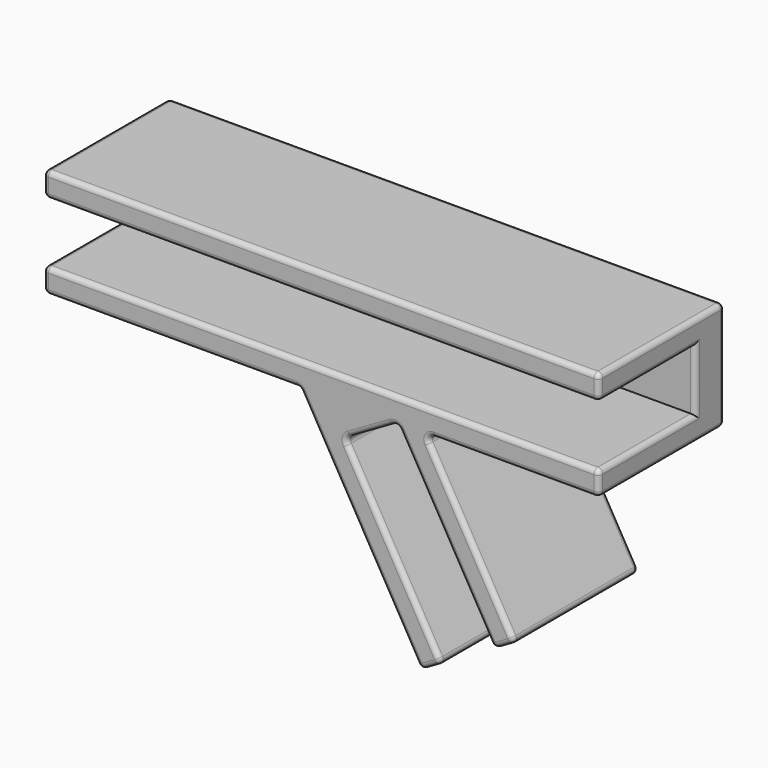
from build123d import *

# Parameters (mm, degrees)
F1_DEPTH      = 12.7
F0_W          = 58.42
F0_H          = 2.54
F0_H_2        = 6.35
F2_DEPTH      = 3.81
F4_T1_DEPTH   = 16.51
F4_T3_DEPTH   = 57.404
F4_T5_DEPTH   = 12.192
F4_T7_DEPTH   = 13.97
F4_T9_DEPTH   = 19.05
F4_T11_DEPTH  = 12.192
F4_T13_DEPTH  = 1.524
F4_T15_DEPTH  = 15.494
F4_T17_DEPTH  = 3.302
F4_T19_DEPTH  = 6.35
F4_T21_DEPTH  = 3.302
F4_T23_DEPTH  = 3.302
F4_T25_DEPTH  = 19.177
F4_T27_DEPTH  = 5.08
F4_T29_DEPTH  = 19.177
F4_T31_DEPTH  = 6.35
F4_S35_W      = 0.508
F4_S35_H      = 0.508
F4_T36_DEPTH  = 0.508
F4_S41_W      = 0.508
F4_S41_H      = 0.508
F4_T42_DEPTH  = 0.508
F4_S47_W      = 0.508
F4_S47_H      = 0.508
F4_T48_DEPTH  = 0.508
F4_S53_W      = 0.508
F4_S53_H      = 0.508
F4_T54_DEPTH  = 0.508
F4_S59_W      = 0.508
F4_S59_H      = 0.508
F4_T60_DEPTH  = 0.508
F4_S65_W      = 0.508
F4_S65_H      = 0.508
F4_T66_DEPTH  = 0.508
F4_S71_W      = 0.508
F4_S71_H      = 0.508
F4_T72_DEPTH  = 0.508
F4_S77_W      = 0.508
F4_S77_H      = 0.508
F4_T78_DEPTH  = 0.508
F4_S83_W      = 0.508
F4_S83_H      = 0.508
F4_T84_DEPTH  = 0.508
F4_S89_W      = 0.508
F4_S89_H      = 0.508
F4_T90_DEPTH  = 0.508
F4_T94_ANGLE  = 90
F4_T96_ANGLE  = 90
F4_T101_DEPTH = 13.462
F4_T105_DEPTH = 7.62
F4_T112_DEPTH = 13.462
F4_T116_DEPTH = 7.62
F4_T123_DEPTH = 13.462
F4_T127_DEPTH = 7.62
F4_T134_DEPTH = 7.62
F4_T138_DEPTH = 13.462
F4_T145_DEPTH = 13.462
F4_T149_DEPTH = 7.62
F4_T156_DEPTH = 13.462
F4_T160_DEPTH = 7.62
F4_T163_DEPTH = 26.130035698
F4_T165_DEPTH = 24.5987060633
F4_T167_DEPTH = 17.4130046129
F4_T169_DEPTH = 16.9025614013
F4_T174_DEPTH = 0.508
F4_S179_W     = 0.508
F4_S179_H     = 0.508
F4_T180_DEPTH = 0.508
F4_S185_W     = 0.508
F4_S185_H     = 0.508
F4_T186_DEPTH = 0.508
F4_T192_DEPTH = 0.508
F4_S197_W     = 0.508
F4_S197_H     = 0.508
F4_T198_DEPTH = 0.508
F4_T204_DEPTH = 0.508
F4_T210_DEPTH = 0.508
F4_S215_W     = 0.508
F4_S215_H     = 0.508
F4_T216_DEPTH = 0.508
F4_T220_ANGLE = 60
F4_T222_ANGLE = 120
F4_T224_ANGLE = 120
F4_T226_ANGLE = 60


# Not quite as in the source:
# - a fillet or chamfer that OpenCascade refuses, or shapes differently, is made with other operations: its cross-section is extruded or revolved along the edge and cut away or added


with BuildPart() as f1:
    # F0 (on Front) → F1 (new body)
    with BuildSketch(Plane.XZ):
        with BuildLine():
            Line((29.21, -5.715), (29.21, -3.175))
            Line((29.21, -3.175), (-29.21, -3.175))
            Line((-29.21, -3.175), (-29.21, -5.715))
            Line((-29.21, -5.715), (-2.2786703653, -5.715))
            Line((-2.2786703653, -5.715), (10.4213296347, -27.7120452561))
            Line((10.4213296347, -27.7120452561), (12.6210341604, -26.4420452561))
            Line((12.6210341604, -26.4420452561), (2.7785341604, -9.3943351826))
            ThreePointArc((2.7785341604, -9.3943351826), (2.7150973921, -8.912485089), (3.0109602918, -8.5269090512))
            Line((3.0109602918, -8.5269090512), (7.410369343, -5.9869090512))
            ThreePointArc((7.410369343, -5.9869090512), (7.8922194366, -5.9234722829), (8.2777954744, -6.2193351826))
            Line((8.2777954744, -6.2193351826), (18.1202954744, -23.2670452561))
            Line((18.1202954744, -23.2670452561), (20.32, -21.9970452561))
            Line((20.32, -21.9970452561), (10.9195567884, -5.715))
            Line((10.9195567884, -5.715), (29.21, -5.715))
        make_face()
    extrude(amount=F1_DEPTH)



with BuildPart() as f1b:
    # F0 (on Front) → F1, piece 2 (new body)
    with BuildSketch(Plane.XZ):
        with Locations((0, 4.445)):
            Rectangle(F0_W, F0_H)
    extrude(amount=F1_DEPTH)


with BuildPart() as f1_1:
    add(f1.part)

    add(f1b.part)  # F2 merges F1b
    # F0 (on Front) → F2 (join)
    with BuildSketch(Plane.XZ):
        with Locations((0, 4.445)):
            Rectangle(F0_W, F0_H)
        Rectangle(F0_W, F0_H_2)
        with BuildLine():
            Line((12.6210341604, -26.4420452561), (18.1202954744, -23.2670452561))
            Line((18.1202954744, -23.2670452561), (8.2777954744, -6.2193351826))
            ThreePointArc((8.2777954744, -6.2193351826), (7.8922194366, -5.9234722829), (7.410369343, -5.9869090512))
            Line((7.410369343, -5.9869090512), (3.0109602918, -8.5269090512))
            ThreePointArc((3.0109602918, -8.5269090512), (2.7150973921, -8.912485089), (2.7785341604, -9.3943351826))
            Line((2.7785341604, -9.3943351826), (12.6210341604, -26.4420452561))
        make_face()
        with BuildLine():
            Line((29.21, -5.715), (29.21, -3.175))
            Line((29.21, -3.175), (-29.21, -3.175))
            Line((-29.21, -3.175), (-29.21, -5.715))
            Line((-29.21, -5.715), (-2.2786703653, -5.715))
            Line((-2.2786703653, -5.715), (10.4213296347, -27.7120452561))
            Line((10.4213296347, -27.7120452561), (12.6210341604, -26.4420452561))
            Line((12.6210341604, -26.4420452561), (2.7785341604, -9.3943351826))
            ThreePointArc((2.7785341604, -9.3943351826), (2.7150973921, -8.912485089), (3.0109602918, -8.5269090512))
            Line((3.0109602918, -8.5269090512), (7.410369343, -5.9869090512))
            ThreePointArc((7.410369343, -5.9869090512), (7.8922194366, -5.9234722829), (8.2777954744, -6.2193351826))
            Line((8.2777954744, -6.2193351826), (18.1202954744, -23.2670452561))
            Line((18.1202954744, -23.2670452561), (20.32, -21.9970452561))
            Line((20.32, -21.9970452561), (10.9195567884, -5.715))
            Line((10.9195567884, -5.715), (29.21, -5.715))
        make_face()
    extrude(amount=-F2_DEPTH)

    # F3: union 

    # F4: fillet of radius 0.508 on 43 edges, made by hand

    # F4_s2 → F4_t1 (join)
    with BuildSketch(Plane.XZ.offset(-3.81)):
        with BuildLine():
            ThreePointArc((11.7994385987, -5.715), (11.3594976935, -5.969), (11.3594976935, -6.477))
            Line((11.3594976935, -6.477), (10.9195567884, -5.715))
            Line((10.9195567884, -5.715), (11.7994385987, -5.715))
        make_face()
        with BuildLine():
            ThreePointArc((-2.1320233969, -5.969), (-2.317964302, -5.7830590949), (-2.571964302, -5.715))
            Line((-2.571964302, -5.715), (-2.2786703653, -5.715))
            Line((-2.2786703653, -5.715), (-2.1320233969, -5.969))
        make_face()
    extrude(amount=F4_T1_DEPTH)

    # F4_s4 → F4_t3 (cut)
    with BuildSketch(Plane.YZ.offset(-28.702)):
        with BuildLine():
            ThreePointArc((3.302, 5.715), (3.6612102448, 5.5662102448), (3.81, 5.207))
            Line((3.81, 5.207), (3.81, 5.715))
            Line((3.81, 5.715), (3.302, 5.715))
        make_face()
        with BuildLine():
            ThreePointArc((-12.7, 5.207), (-12.5512102448, 5.5662102448), (-12.192, 5.715))
            Line((-12.192, 5.715), (-12.7, 5.715))
            Line((-12.7, 5.715), (-12.7, 5.207))
        make_face()
        with BuildLine():
            ThreePointArc((-12.192, 3.175), (-12.5512102448, 3.3237897552), (-12.7, 3.683))
            Line((-12.7, 3.683), (-12.7, 3.175))
            Line((-12.7, 3.175), (-12.192, 3.175))
        make_face()
        with BuildLine():
            ThreePointArc((-12.192, -3.175), (-12.5512102448, -3.3237897552), (-12.7, -3.683))
            Line((-12.7, -3.683), (-12.7, -3.175))
            Line((-12.7, -3.175), (-12.192, -3.175))
        make_face()
    extrude(amount=F4_T3_DEPTH, mode=Mode.SUBTRACT)

    # F4_s6 → F4_t5 (cut)
    with BuildSketch(Plane.XY.offset(-6.985)):
        with BuildLine():
            ThreePointArc((-29.21, 3.302), (-29.0612102448, 3.6612102448), (-28.702, 3.81))
            Line((-28.702, 3.81), (-29.21, 3.81))
            Line((-29.21, 3.81), (-29.21, 3.302))
        make_face()
        with BuildLine():
            ThreePointArc((29.21, 3.302), (29.0612102448, 3.6612102448), (28.702, 3.81))
            Line((28.702, 3.81), (29.21, 3.81))
            Line((29.21, 3.81), (29.21, 3.302))
        make_face()
    extrude(amount=F4_T5_DEPTH, mode=Mode.SUBTRACT)

    # F4_s8 → F4_t7 (cut)
    with BuildSketch(Plane(origin=(-5.2835226281, 0, -3.0504432116), x_dir=(0, 1, 0), z_dir=(0.8660254038, 0, 0.5))):
        with BuildLine():
            ThreePointArc((3.81, -28.702), (3.6612102448, -29.0612102448), (3.302, -29.21))
            Line((3.302, -29.21), (3.81, -29.21))
            Line((3.81, -29.21), (3.81, -28.702))
        make_face()
    extrude(amount=F4_T7_DEPTH, mode=Mode.SUBTRACT)

    # F4_s10 → F4_t9 (cut)
    with BuildSketch(Plane.XZ.offset(-5.08)):
        with BuildLine():
            ThreePointArc((19.8800590949, -22.2510452561), (20.1167494146, -21.9425844259), (20.066, -21.557104351))
            Line((20.066, -21.557104351), (20.32, -21.9970452561))
            Line((20.32, -21.9970452561), (19.8800590949, -22.2510452561))
        make_face()
        with BuildLine():
            ThreePointArc((29.21, -5.207), (29.0612102448, -5.5662102448), (28.702, -5.715))
            Line((28.702, -5.715), (29.21, -5.715))
            Line((29.21, -5.715), (29.21, -5.207))
        make_face()
        with BuildLine():
            ThreePointArc((-29.21, -5.207), (-29.0612102448, -5.5662102448), (-28.702, -5.715))
            Line((-28.702, -5.715), (-29.21, -5.715))
            Line((-29.21, -5.715), (-29.21, -5.207))
        make_face()
        with BuildLine():
            ThreePointArc((10.8612705399, -27.4580452561), (10.475790465, -27.5087946708), (10.1673296347, -27.272104351))
            Line((10.1673296347, -27.272104351), (10.4213296347, -27.7120452561))
            Line((10.4213296347, -27.7120452561), (10.8612705399, -27.4580452561))
        make_face()
    extrude(amount=F4_T9_DEPTH, mode=Mode.SUBTRACT)

    # F4_s12 → F4_t11 (cut)
    with BuildSketch(Plane.XZ):
        with BuildLine():
            ThreePointArc((28.702, 3.175), (29.0612102448, 3.3237897552), (29.21, 3.683))
            Line((29.21, 3.683), (29.21, 3.175))
            Line((29.21, 3.175), (28.702, 3.175))
        make_face()
        with BuildLine():
            ThreePointArc((29.21, -3.683), (29.0612102448, -3.3237897552), (28.702, -3.175))
            Line((28.702, -3.175), (29.21, -3.175))
            Line((29.21, -3.175), (29.21, -3.683))
        make_face()
        with BuildLine():
            ThreePointArc((-28.702, 3.175), (-29.0612102448, 3.3237897552), (-29.21, 3.683))
            Line((-29.21, 3.683), (-29.21, 3.175))
            Line((-29.21, 3.175), (-28.702, 3.175))
        make_face()
        with BuildLine():
            ThreePointArc((-29.21, -3.683), (-29.0612102448, -3.3237897552), (-28.702, -3.175))
            Line((-28.702, -3.175), (-29.21, -3.175))
            Line((-29.21, -3.175), (-29.21, -3.683))
        make_face()
        with BuildLine():
            ThreePointArc((18.5602363795, -23.0130452561), (18.1747563046, -23.0637946708), (17.8662954744, -22.827104351))
            Line((17.8662954744, -22.827104351), (18.1202954744, -23.2670452561))
            Line((18.1202954744, -23.2670452561), (18.5602363795, -23.0130452561))
        make_face()
        with BuildLine():
            ThreePointArc((12.1810932552, -26.6960452561), (12.417783575, -26.3875844259), (12.3670341604, -26.002104351))
            Line((12.3670341604, -26.002104351), (12.6210341604, -26.4420452561))
            Line((12.6210341604, -26.4420452561), (12.1810932552, -26.6960452561))
        make_face()
    extrude(amount=F4_T11_DEPTH, mode=Mode.SUBTRACT)

    # F4_s14 → F4_t13 (cut)
    with BuildSketch(Plane.XY.offset(3.683)):
        with BuildLine():
            ThreePointArc((29.21, -12.192), (29.0612102448, -12.5512102448), (28.702, -12.7))
            Line((28.702, -12.7), (29.21, -12.7))
            Line((29.21, -12.7), (29.21, -12.192))
        make_face()
        with BuildLine():
            ThreePointArc((-29.21, -12.192), (-29.0612102448, -12.5512102448), (-28.702, -12.7))
            Line((-28.702, -12.7), (-29.21, -12.7))
            Line((-29.21, -12.7), (-29.21, -12.192))
        make_face()
    extrude(amount=F4_T13_DEPTH, mode=Mode.SUBTRACT)

    # F4_s16 → F4_t15 (cut)
    with BuildSketch(Plane.XZ.offset(-3.302)):
        with BuildLine():
            ThreePointArc((29.21, 5.207), (29.0612102448, 5.5662102448), (28.702, 5.715))
            Line((28.702, 5.715), (29.21, 5.715))
            Line((29.21, 5.715), (29.21, 5.207))
        make_face()
        with BuildLine():
            ThreePointArc((-29.21, 5.207), (-29.0612102448, 5.5662102448), (-28.702, 5.715))
            Line((-28.702, 5.715), (-29.21, 5.715))
            Line((-29.21, 5.715), (-29.21, 5.207))
        make_face()
    extrude(amount=F4_T15_DEPTH, mode=Mode.SUBTRACT)

    # F4_s18 → F4_t17 (cut)
    with BuildSketch(Plane.XY.offset(-6.985)):
        with BuildLine():
            ThreePointArc((29.21, -12.192), (29.0612102448, -12.5512102448), (28.702, -12.7))
            Line((28.702, -12.7), (29.21, -12.7))
            Line((29.21, -12.7), (29.21, -12.192))
        make_face()
        with BuildLine():
            ThreePointArc((-29.21, -12.192), (-29.0612102448, -12.5512102448), (-28.702, -12.7))
            Line((-28.702, -12.7), (-29.21, -12.7))
            Line((-29.21, -12.7), (-29.21, -12.192))
        make_face()
    extrude(amount=F4_T17_DEPTH, mode=Mode.SUBTRACT)

    # F4_s20 → F4_t19 (cut)
    with BuildSketch(Plane.XY.offset(-3.175)):
        with BuildLine():
            ThreePointArc((29.21, 0.508), (29.0612102448, 0.1487897552), (28.702, 0))
            Line((28.702, 0), (29.21, 0))
            Line((29.21, 0), (29.21, 0.508))
        make_face()
        with BuildLine():
            ThreePointArc((-29.21, 0.508), (-29.0612102448, 0.1487897552), (-28.702, 0))
            Line((-28.702, 0), (-29.21, 0))
            Line((-29.21, 0), (-29.21, 0.508))
        make_face()
    extrude(amount=F4_T19_DEPTH, mode=Mode.SUBTRACT)

    # F4_s22 → F4_t21 (cut)
    with BuildSketch(Plane(origin=(3.9552363795, 0, 2.2835567884), x_dir=(0, 1, 0), z_dir=(0.8660254038, 0, 0.5))):
        with BuildLine():
            ThreePointArc((-12.7, -28.702), (-12.5512102448, -29.0612102448), (-12.192, -29.21))
            Line((-12.192, -29.21), (-12.7, -29.21))
            Line((-12.7, -29.21), (-12.7, -28.702))
        make_face()
    extrude(amount=F4_T21_DEPTH, mode=Mode.SUBTRACT)

    # F4_s24 → F4_t23 (cut)
    with BuildSketch(Plane(origin=(-5.2835226281, 0, -3.0504432116), x_dir=(0, 1, 0), z_dir=(0.8660254038, 0, 0.5))):
        with BuildLine():
            ThreePointArc((-12.7, -28.702), (-12.5512102448, -29.0612102448), (-12.192, -29.21))
            Line((-12.192, -29.21), (-12.7, -29.21))
            Line((-12.7, -29.21), (-12.7, -28.702))
        make_face()
    extrude(amount=F4_T23_DEPTH, mode=Mode.SUBTRACT)

    # F4_s26 → F4_t25 (cut)
    with BuildSketch(Plane(origin=(14.351, 0, -24.8566611394), x_dir=(0, 1, 0), z_dir=(-0.5, 0, 0.8660254038))):
        with BuildLine():
            ThreePointArc((-12.7, 2.7988864232), (-12.5512102448, 2.4396761783), (-12.192, 2.2908864232))
            Line((-12.192, 2.2908864232), (-12.7, 2.2908864232))
            Line((-12.7, 2.2908864232), (-12.7, 2.7988864232))
        make_face()
    extrude(amount=F4_T25_DEPTH, mode=Mode.SUBTRACT)

    # F4_s28 → F4_t27 (cut)
    with BuildSketch(Plane(origin=(-1.4340397082, 0, -0.8279432116), x_dir=(0, 1, 0), z_dir=(0.8660254038, 0, 0.5))):
        with BuildLine():
            ThreePointArc((-12.7, -8.382), (-12.5512102448, -8.7412102448), (-12.192, -8.89))
            Line((-12.192, -8.89), (-12.7, -8.89))
            Line((-12.7, -8.89), (-12.7, -8.382))
        make_face()
    extrude(amount=F4_T27_DEPTH, mode=Mode.SUBTRACT)

    # F4_s30 → F4_t29 (cut)
    with BuildSketch(Plane(origin=(4.7625, 0, -8.248891971), x_dir=(0, 1, 0), z_dir=(0.5, 0, -0.8660254038))):
        with BuildLine():
            ThreePointArc((-12.7, 4.5671135768), (-12.5512102448, 4.207903332), (-12.192, 4.0591135768))
            Line((-12.192, 4.0591135768), (-12.7, 4.0591135768))
            Line((-12.7, 4.0591135768), (-12.7, 4.5671135768))
        make_face()
    extrude(amount=F4_T29_DEPTH, mode=Mode.SUBTRACT)

    # F4_s32 → F4_t31 (cut)
    with BuildSketch(Plane(origin=(-1.9839658396, 0, -1.1454432116), x_dir=(0, 1, 0), z_dir=(0.8660254038, 0, 0.5))):
        with BuildLine():
            ThreePointArc((0.508, -29.21), (0.1487897552, -29.0612102448), (0, -28.702))
            Line((0, -28.702), (0, -29.21))
            Line((0, -29.21), (0.508, -29.21))
        make_face()
    extrude(amount=F4_T31_DEPTH, mode=Mode.SUBTRACT)


with BuildPart() as f4_tool34:
    # F4_s35 → F4_t36 (new body)
    with BuildSketch(Plane.XZ.offset(-3.302)):
        with Locations((28.956, 5.461)):
            Rectangle(F4_S35_W, F4_S35_H)
    extrude(amount=-F4_T36_DEPTH)

    # F4_s37 → F4_t38 (revolve, cut)
    with BuildSketch(Plane(origin=(28.702, 3.302, 5.207), x_dir=(-0.7071067812, 0, -0.7071067812), z_dir=(0.7071067812, 0, -0.7071067812))):
        with BuildLine():
            ThreePointArc((0, -0.508), (0.508, 0), (0, 0.508))
            Line((0, 0.508), (0, -0.508))
        make_face()
    revolve(axis=Axis((28.702, 3.302, 5.207), (0, 1, 0)), mode=Mode.SUBTRACT)


with BuildPart() as f1_2:
    add(f1_1.part)

    # F4_t33: cut F4_tool34
    add(f4_tool34.part, mode=Mode.SUBTRACT)


with BuildPart() as f4_tool40:
    # F4_s41 → F4_t42 (new body)
    with BuildSketch(Plane.XZ.offset(-3.302)):
        with Locations((-28.956, 5.461)):
            Rectangle(F4_S41_W, F4_S41_H)
    extrude(amount=-F4_T42_DEPTH)

    # F4_s43 → F4_t44 (revolve, cut)
    with BuildSketch(Plane(origin=(-28.702, 3.302, 5.207), x_dir=(0.7071067812, 0, -0.7071067812), z_dir=(0.7071067812, 0, 0.7071067812))):
        with BuildLine():
            ThreePointArc((0, -0.508), (0.508, 0), (0, 0.508))
            Line((0, 0.508), (0, -0.508))
        make_face()
    revolve(axis=Axis((-28.702, 3.302, 5.207), (0, 1, 0)), mode=Mode.SUBTRACT)


with BuildPart() as f1_3:
    add(f1_2.part)

    # F4_t39: cut F4_tool40
    add(f4_tool40.part, mode=Mode.SUBTRACT)


with BuildPart() as f4_tool46:
    # F4_s47 → F4_t48 (new body)
    with BuildSketch(Plane.XY.offset(3.683)):
        with Locations((28.956, -12.446)):
            Rectangle(F4_S47_W, F4_S47_H)
    extrude(amount=-F4_T48_DEPTH)

    # F4_s49 → F4_t50 (revolve, cut)
    with BuildSketch(Plane(origin=(28.702, -12.192, 3.683), x_dir=(-0.7071067812, 0.7071067812, 0), z_dir=(-0.7071067812, -0.7071067812, 0))):
        with BuildLine():
            ThreePointArc((0, -0.508), (0.508, 0), (0, 0.508))
            Line((0, 0.508), (0, -0.508))
        make_face()
    revolve(axis=Axis((28.702, -12.192, 3.683), (0, 0, -1)), mode=Mode.SUBTRACT)


with BuildPart() as f1_4:
    add(f1_3.part)

    # F4_t45: cut F4_tool46
    add(f4_tool46.part, mode=Mode.SUBTRACT)


with BuildPart() as f4_tool52:
    # F4_s53 → F4_t54 (new body)
    with BuildSketch(Plane.YZ.offset(28.702)):
        with Locations((-12.446, 5.461)):
            Rectangle(F4_S53_W, F4_S53_H)
    extrude(amount=F4_T54_DEPTH)

    # F4_s55 → F4_t56 (revolve, cut)
    with BuildSketch(Plane(origin=(28.702, -12.192, 5.207), x_dir=(0, 0.7071067812, -0.7071067812), z_dir=(0, -0.7071067812, -0.7071067812))):
        with BuildLine():
            ThreePointArc((0, -0.508), (0.508, 0), (0, 0.508))
            Line((0, 0.508), (0, -0.508))
        make_face()
    revolve(axis=Axis((28.702, -12.192, 5.207), (1, 0, 0)), mode=Mode.SUBTRACT)


with BuildPart() as f1_5:
    add(f1_4.part)

    # F4_t51: cut F4_tool52
    add(f4_tool52.part, mode=Mode.SUBTRACT)


with BuildPart() as f4_tool58:
    # F4_s59 → F4_t60 (new body)
    with BuildSketch(Plane.YZ.offset(28.702)):
        with Locations((-12.446, -3.429)):
            Rectangle(F4_S59_W, F4_S59_H)
    extrude(amount=F4_T60_DEPTH)

    # F4_s61 → F4_t62 (revolve, cut)
    with BuildSketch(Plane(origin=(28.702, -12.192, -3.683), x_dir=(0, 0.7071067812, -0.7071067812), z_dir=(0, -0.7071067812, -0.7071067812))):
        with BuildLine():
            ThreePointArc((0, -0.508), (0.508, 0), (0, 0.508))
            Line((0, 0.508), (0, -0.508))
        make_face()
    revolve(axis=Axis((28.702, -12.192, -3.683), (1, 0, 0)), mode=Mode.SUBTRACT)


with BuildPart() as f1_6:
    add(f1_5.part)

    # F4_t57: cut F4_tool58
    add(f4_tool58.part, mode=Mode.SUBTRACT)


with BuildPart() as f4_tool64:
    # F4_s65 → F4_t66 (new body)
    with BuildSketch(Plane.YZ.offset(-28.702)):
        with Locations((-12.446, 5.461)):
            Rectangle(F4_S65_W, F4_S65_H)
    extrude(amount=-F4_T66_DEPTH)

    # F4_s67 → F4_t68 (revolve, cut)
    with BuildSketch(Plane(origin=(-28.702, -12.192, 5.207), x_dir=(0, 0.7071067812, -0.7071067812), z_dir=(0, 0.7071067812, 0.7071067812))):
        with BuildLine():
            ThreePointArc((0, -0.508), (0.508, 0), (0, 0.508))
            Line((0, 0.508), (0, -0.508))
        make_face()
    revolve(axis=Axis((-28.702, -12.192, 5.207), (-1, 0, 0)), mode=Mode.SUBTRACT)


with BuildPart() as f1_7:
    add(f1_6.part)

    # F4_t63: cut F4_tool64
    add(f4_tool64.part, mode=Mode.SUBTRACT)


with BuildPart() as f4_tool70:
    # F4_s71 → F4_t72 (new body)
    with BuildSketch(Plane.XY.offset(3.683)):
        with Locations((-28.956, -12.446)):
            Rectangle(F4_S71_W, F4_S71_H)
    extrude(amount=-F4_T72_DEPTH)

    # F4_s73 → F4_t74 (revolve, cut)
    with BuildSketch(Plane(origin=(-28.702, -12.192, 3.683), x_dir=(0.7071067812, 0.7071067812, 0), z_dir=(-0.7071067812, 0.7071067812, 0))):
        with BuildLine():
            ThreePointArc((0, -0.508), (0.508, 0), (0, 0.508))
            Line((0, 0.508), (0, -0.508))
        make_face()
    revolve(axis=Axis((-28.702, -12.192, 3.683), (0, 0, -1)), mode=Mode.SUBTRACT)


with BuildPart() as f1_8:
    add(f1_7.part)

    # F4_t69: cut F4_tool70
    add(f4_tool70.part, mode=Mode.SUBTRACT)


with BuildPart() as f4_tool76:
    # F4_s77 → F4_t78 (new body)
    with BuildSketch(Plane(origin=(3.9552363795, 0, 2.2835567884), x_dir=(0, 1, 0), z_dir=(-0.8660254038, 0, -0.5))):
        with Locations((-12.446, 28.956)):
            Rectangle(F4_S77_W, F4_S77_H)
    extrude(amount=F4_T78_DEPTH)

    # F4_s79 → F4_t80 (revolve, cut)
    with BuildSketch(Plane(origin=(18.3062363795, -12.192, -22.573104351), x_dir=(-0.3535533906, 0.7071067812, 0.6123724357), z_dir=(-0.3535533906, -0.7071067812, 0.6123724357))):
        with BuildLine():
            ThreePointArc((0, -0.508), (0.508, 0), (0, 0.508))
            Line((0, 0.508), (0, -0.508))
        make_face()
    revolve(axis=Axis((18.3062363795, -12.192, -22.573104351), (-0.8660254038, 0, -0.5)), mode=Mode.SUBTRACT)


with BuildPart() as f1_9:
    add(f1_8.part)

    # F4_t75: cut F4_tool76
    add(f4_tool76.part, mode=Mode.SUBTRACT)


with BuildPart() as f4_tool82:
    # F4_s83 → F4_t84 (new body)
    with BuildSketch(Plane.YZ.offset(-28.702)):
        with Locations((-12.446, -3.429)):
            Rectangle(F4_S83_W, F4_S83_H)
    extrude(amount=-F4_T84_DEPTH)

    # F4_s85 → F4_t86 (revolve, cut)
    with BuildSketch(Plane(origin=(-28.702, -12.192, -3.683), x_dir=(0, 0.7071067812, -0.7071067812), z_dir=(0, 0.7071067812, 0.7071067812))):
        with BuildLine():
            ThreePointArc((0, -0.508), (0.508, 0), (0, 0.508))
            Line((0, 0.508), (0, -0.508))
        make_face()
    revolve(axis=Axis((-28.702, -12.192, -3.683), (-1, 0, 0)), mode=Mode.SUBTRACT)


with BuildPart() as f1_10:
    add(f1_9.part)

    # F4_t81: cut F4_tool82
    add(f4_tool82.part, mode=Mode.SUBTRACT)


with BuildPart() as f4_tool88:
    # F4_s89 → F4_t90 (new body)
    with BuildSketch(Plane(origin=(14.351, 0, -24.8566611394), x_dir=(0, 1, 0), z_dir=(0.5, 0, -0.8660254038))):
        with Locations((-12.446, -2.5448864232)):
            Rectangle(F4_S89_W, F4_S89_H)
    extrude(amount=F4_T90_DEPTH)

    # F4_s91 → F4_t92 (revolve, cut)
    with BuildSketch(Plane(origin=(11.9270932552, -12.192, -26.256104351), x_dir=(-0.6123724357, 0.7071067812, -0.3535533906), z_dir=(-0.6123724357, -0.7071067812, -0.3535533906))):
        with BuildLine():
            ThreePointArc((0, -0.508), (0.508, 0), (0, 0.508))
            Line((0, 0.508), (0, -0.508))
        make_face()
    revolve(axis=Axis((11.9270932552, -12.192, -26.256104351), (0.5, 0, -0.8660254038)), mode=Mode.SUBTRACT)


with BuildPart() as f1_11:
    add(f1_10.part)

    # F4_t87: cut F4_tool88
    add(f4_tool88.part, mode=Mode.SUBTRACT)

    # F4_s93 → F4_t94 (revolve, cut)
    with BuildSketch(Plane(origin=(4.7625, 0, -8.248891971), x_dir=(0, 1, 0), z_dir=(0.5, 0, -0.8660254038))):
        with BuildLine():
            ThreePointArc((-12.7, -2.7988864232), (-12.5512102448, -2.4396761783), (-12.192, -2.2908864232))
            Line((-12.192, -2.2908864232), (-12.7, -2.2908864232))
            Line((-12.7, -2.2908864232), (-12.7, -2.7988864232))
        make_face()
    revolve(axis=Axis((3.3284602918, -12.7, -9.0768351826), (0, 1, 0)), revolution_arc=F4_T94_ANGLE, mode=Mode.SUBTRACT)

    # F4_s95 → F4_t96 (revolve, cut)
    with BuildSketch(Plane(origin=(2.965369343, 0, 1.7120567884), x_dir=(0, 1, 0), z_dir=(-0.8660254038, 0, -0.5))):
        with BuildLine():
            ThreePointArc((-12.7, 8.382), (-12.5512102448, 8.7412102448), (-12.192, 8.89))
            Line((-12.192, 8.89), (-12.7, 8.89))
            Line((-12.7, 8.89), (-12.7, 8.382))
        make_face()
    revolve(axis=Axis((7.727869343, -12.7, -6.5368351826), (0, 1, 0)), revolution_arc=F4_T96_ANGLE, mode=Mode.SUBTRACT)


with BuildPart() as f4_tool99:
    # F4_s100 → F4_t101 (new body)
    with BuildSketch(Plane.XZ.offset(-1.27)):
        with BuildLine():
            ThreePointArc((28.702, 3.175), (29.0612102448, 3.3237897552), (29.21, 3.683))
            Line((29.21, 3.683), (29.21, 3.175))
            Line((29.21, 3.175), (28.702, 3.175))
        make_face()
    extrude(amount=F4_T101_DEPTH)

    split(bisect_by=Plane.XZ, keep=Keep.BOTTOM)


with BuildPart() as f4_tool103:
    # F4_s104 → F4_t105 (new body)
    with BuildSketch(Plane.XY.offset(-3.175)):
        with BuildLine():
            ThreePointArc((29.21, 0.508), (29.0612102448, 0.1487897552), (28.702, 0))
            Line((28.702, 0), (29.21, 0))
            Line((29.21, 0), (29.21, 0.508))
        make_face()
    extrude(amount=F4_T105_DEPTH)

    split(bisect_by=Plane.XY.offset(3.175), keep=Keep.TOP)


with BuildPart() as f4_tool99_1:
    add(f4_tool99.part)

    # F4_t107: intersect F4_tool103
    add(f4_tool103.part, mode=Mode.INTERSECT)


with BuildPart() as f1_12:
    add(f1_11.part)

    # F4_t97: cut F4_tool99
    add(f4_tool99_1.part, mode=Mode.SUBTRACT)


with BuildPart() as f4_tool110:
    # F4_s111 → F4_t112 (new body)
    with BuildSketch(Plane.XZ.offset(-1.27)):
        with BuildLine():
            ThreePointArc((29.21, -3.683), (29.0612102448, -3.3237897552), (28.702, -3.175))
            Line((28.702, -3.175), (29.21, -3.175))
            Line((29.21, -3.175), (29.21, -3.683))
        make_face()
    extrude(amount=F4_T112_DEPTH)

    split(bisect_by=Plane.XZ, keep=Keep.BOTTOM)


with BuildPart() as f4_tool114:
    # F4_s115 → F4_t116 (new body)
    with BuildSketch(Plane.XY.offset(-4.445)):
        with BuildLine():
            ThreePointArc((29.21, 0.508), (29.0612102448, 0.1487897552), (28.702, 0))
            Line((28.702, 0), (29.21, 0))
            Line((29.21, 0), (29.21, 0.508))
        make_face()
    extrude(amount=F4_T116_DEPTH)

    split(bisect_by=Plane.XY.offset(-3.175), keep=Keep.BOTTOM)


with BuildPart() as f4_tool110_1:
    add(f4_tool110.part)

    # F4_t118: intersect F4_tool114
    add(f4_tool114.part, mode=Mode.INTERSECT)


with BuildPart() as f1_13:
    add(f1_12.part)

    # F4_t108: cut F4_tool110
    add(f4_tool110_1.part, mode=Mode.SUBTRACT)


with BuildPart() as f4_tool121:
    # F4_s122 → F4_t123 (new body)
    with BuildSketch(Plane.XZ.offset(-1.27)):
        with BuildLine():
            ThreePointArc((-28.702, 3.175), (-29.0612102448, 3.3237897552), (-29.21, 3.683))
            Line((-29.21, 3.683), (-29.21, 3.175))
            Line((-29.21, 3.175), (-28.702, 3.175))
        make_face()
    extrude(amount=F4_T123_DEPTH)

    split(bisect_by=Plane.XZ, keep=Keep.BOTTOM)


with BuildPart() as f4_tool125:
    # F4_s126 → F4_t127 (new body)
    with BuildSketch(Plane.XY.offset(4.445)):
        with BuildLine():
            ThreePointArc((-29.21, 0.508), (-29.0612102448, 0.1487897552), (-28.702, 0))
            Line((-28.702, 0), (-29.21, 0))
            Line((-29.21, 0), (-29.21, 0.508))
        make_face()
    extrude(amount=-F4_T127_DEPTH)

    split(bisect_by=Plane.XY.offset(3.175), keep=Keep.TOP)


with BuildPart() as f4_tool121_1:
    add(f4_tool121.part)

    # F4_t129: intersect F4_tool125
    add(f4_tool125.part, mode=Mode.INTERSECT)


with BuildPart() as f1_14:
    add(f1_13.part)

    # F4_t119: cut F4_tool121
    add(f4_tool121_1.part, mode=Mode.SUBTRACT)


with BuildPart() as f4_tool132:
    # F4_s133 → F4_t134 (new body)
    with BuildSketch(Plane.XY.offset(3.175)):
        with BuildLine():
            ThreePointArc((-29.21, 0.508), (-29.0612102448, 0.1487897552), (-28.702, 0))
            Line((-28.702, 0), (-29.21, 0))
            Line((-29.21, 0), (-29.21, 0.508))
        make_face()
    extrude(amount=-F4_T134_DEPTH)

    split(bisect_by=Plane.XY.offset(-3.175), keep=Keep.BOTTOM)


with BuildPart() as f4_tool136:
    # F4_s137 → F4_t138 (new body)
    with BuildSketch(Plane.XZ.offset(-1.27)):
        with BuildLine():
            ThreePointArc((-29.21, -3.683), (-29.0612102448, -3.3237897552), (-28.702, -3.175))
            Line((-28.702, -3.175), (-29.21, -3.175))
            Line((-29.21, -3.175), (-29.21, -3.683))
        make_face()
    extrude(amount=F4_T138_DEPTH)

    split(bisect_by=Plane.XZ, keep=Keep.BOTTOM)


with BuildPart() as f4_tool132_1:
    add(f4_tool132.part)

    # F4_t140: intersect F4_tool136
    add(f4_tool136.part, mode=Mode.INTERSECT)


with BuildPart() as f1_15:
    add(f1_14.part)

    # F4_t130: cut F4_tool132
    add(f4_tool132_1.part, mode=Mode.SUBTRACT)


with BuildPart() as f4_tool143:
    # F4_s144 → F4_t145 (new body)
    with BuildSketch(Plane.XZ.offset(-1.27)):
        with BuildLine():
            ThreePointArc((18.5602363795, -23.0130452561), (18.1747563046, -23.0637946708), (17.8662954744, -22.827104351))
            Line((17.8662954744, -22.827104351), (18.1202954744, -23.2670452561))
            Line((18.1202954744, -23.2670452561), (18.5602363795, -23.0130452561))
        make_face()
    extrude(amount=F4_T145_DEPTH)

    split(bisect_by=Plane.XZ, keep=Keep.BOTTOM)


with BuildPart() as f4_tool147:
    # F4_s148 → F4_t149 (new body)
    with BuildSketch(Plane(origin=(-1.9839658396, 0, -1.1454432116), x_dir=(0, 1, 0), z_dir=(0.8660254038, 0, 0.5))):
        with BuildLine():
            ThreePointArc((0.508, -29.21), (0.1487897552, -29.0612102448), (0, -28.702))
            Line((0, -28.702), (0, -29.21))
            Line((0, -29.21), (0.508, -29.21))
        make_face()
    extrude(amount=F4_T149_DEPTH)

    split(bisect_by=Plane(origin=(3.5152954744, 0, 2.0295567884), x_dir=(0, 1, 0), z_dir=(0.8660254038, 0, 0.5)), keep=Keep.TOP)


with BuildPart() as f4_tool143_1:
    add(f4_tool143.part)

    # F4_t151: intersect F4_tool147
    add(f4_tool147.part, mode=Mode.INTERSECT)


with BuildPart() as f1_16:
    add(f1_15.part)

    # F4_t141: cut F4_tool143
    add(f4_tool143_1.part, mode=Mode.SUBTRACT)


with BuildPart() as f4_tool154:
    # F4_s155 → F4_t156 (new body)
    with BuildSketch(Plane.XZ.offset(-1.27)):
        with BuildLine():
            ThreePointArc((12.1810932552, -26.6960452561), (12.417783575, -26.3875844259), (12.3670341604, -26.002104351))
            Line((12.3670341604, -26.002104351), (12.6210341604, -26.4420452561))
            Line((12.6210341604, -26.4420452561), (12.1810932552, -26.6960452561))
        make_face()
    extrude(amount=F4_T156_DEPTH)

    split(bisect_by=Plane.XZ, keep=Keep.BOTTOM)


with BuildPart() as f4_tool158:
    # F4_s159 → F4_t160 (new body)
    with BuildSketch(Plane(origin=(-3.0838181024, 0, -1.7804432116), x_dir=(0, 1, 0), z_dir=(0.8660254038, 0, 0.5))):
        with BuildLine():
            ThreePointArc((0.508, -29.21), (0.1487897552, -29.0612102448), (0, -28.702))
            Line((0, -28.702), (0, -29.21))
            Line((0, -29.21), (0.508, -29.21))
        make_face()
    extrude(amount=F4_T160_DEPTH)

    split(bisect_by=Plane(origin=(-1.9839658396, 0, -1.1454432116), x_dir=(0, 1, 0), z_dir=(-0.8660254038, 0, -0.5)), keep=Keep.TOP)


with BuildPart() as f4_tool154_1:
    add(f4_tool154.part)

    # F4_t162: intersect F4_tool158
    add(f4_tool158.part, mode=Mode.INTERSECT)


with BuildPart() as f1_17:
    add(f1_16.part)

    # F4_t152: cut F4_tool154
    add(f4_tool154_1.part, mode=Mode.SUBTRACT)

    # F4_s164 → F4_t163 (cut)
    with BuildSketch(Plane.YZ.offset(-28.702)):
        with BuildLine():
            ThreePointArc((3.81, -5.207), (3.6612102448, -5.5662102448), (3.302, -5.715))
            Line((3.302, -5.715), (3.81, -5.715))
            Line((3.81, -5.715), (3.81, -5.207))
        make_face()
        with BuildLine():
            ThreePointArc((-12.7, -5.207), (-12.5512102448, -5.5662102448), (-12.192, -5.715))
            Line((-12.192, -5.715), (-12.7, -5.715))
            Line((-12.7, -5.715), (-12.7, -5.207))
        make_face()
    extrude(amount=F4_T163_DEPTH, mode=Mode.SUBTRACT)

    # F4_s166 → F4_t165 (cut)
    with BuildSketch(Plane(origin=(2.0516469684, 0, -3.5535567884), x_dir=(0, 1, 0), z_dir=(0.5, 0, -0.8660254038))):
        with BuildLine():
            ThreePointArc((3.81, -4.3228864232), (3.6612102448, -4.682096668), (3.302, -4.8308864232))
            Line((3.302, -4.8308864232), (3.81, -4.8308864232))
            Line((3.81, -4.8308864232), (3.81, -4.3228864232))
        make_face()
        with BuildLine():
            ThreePointArc((-12.7, -4.3228864232), (-12.5512102448, -4.682096668), (-12.192, -4.8308864232))
            Line((-12.192, -4.8308864232), (-12.7, -4.8308864232))
            Line((-12.7, -4.8308864232), (-12.7, -4.3228864232))
        make_face()
    extrude(amount=F4_T165_DEPTH, mode=Mode.SUBTRACT)

    # F4_s168 → F4_t167 (cut)
    with BuildSketch(Plane(origin=(14.351, 0, -24.8566611394), x_dir=(0, 1, 0), z_dir=(-0.5, 0, 0.8660254038))):
        with BuildLine():
            ThreePointArc((3.81, -6.0911135768), (3.6612102448, -6.4503238217), (3.302, -6.5991135768))
            Line((3.302, -6.5991135768), (3.81, -6.5991135768))
            Line((3.81, -6.5991135768), (3.81, -6.0911135768))
        make_face()
        with BuildLine():
            ThreePointArc((-12.7, -6.0911135768), (-12.5512102448, -6.4503238217), (-12.192, -6.5991135768))
            Line((-12.192, -6.5991135768), (-12.7, -6.5991135768))
            Line((-12.7, -6.5991135768), (-12.7, -6.0911135768))
        make_face()
    extrude(amount=F4_T167_DEPTH, mode=Mode.SUBTRACT)

    # F4_s170 → F4_t169 (cut)
    with BuildSketch(Plane.YZ.offset(11.7994385987)):
        with BuildLine():
            ThreePointArc((3.81, -5.207), (3.6612102448, -5.5662102448), (3.302, -5.715))
            Line((3.302, -5.715), (3.81, -5.715))
            Line((3.81, -5.715), (3.81, -5.207))
        make_face()
        with BuildLine():
            ThreePointArc((-12.7, -5.207), (-12.5512102448, -5.5662102448), (-12.192, -5.715))
            Line((-12.192, -5.715), (-12.7, -5.715))
            Line((-12.7, -5.715), (-12.7, -5.207))
        make_face()
    extrude(amount=F4_T169_DEPTH, mode=Mode.SUBTRACT)


with BuildPart() as f4_tool172:
    # F4_s173 → F4_t174 (new body)
    with BuildSketch(Plane.XZ.offset(12.192)):
        Polygon((10.6072705399, -27.018104351), (10.1673296347, -27.272104351), (10.4213296347, -27.7120452561), (10.8612705399, -27.4580452561), align=None)
    extrude(amount=F4_T174_DEPTH)

    # F4_s175 → F4_t176 (revolve, cut)
    with BuildSketch(Plane(origin=(10.6072705399, -12.192, -27.018104351), x_dir=(0.2588190451, 0, 0.9659258263), z_dir=(0.9659258263, 0, -0.2588190451))):
        with BuildLine():
            ThreePointArc((0, -0.508), (0.508, 0), (0, 0.508))
            Line((0, 0.508), (0, -0.508))
        make_face()
    revolve(axis=Axis((10.6072705399, -12.192, -27.018104351), (0, -1, 0)), mode=Mode.SUBTRACT)


with BuildPart() as f1_18:
    add(f1_17.part)

    # F4_t171: cut F4_tool172
    add(f4_tool172.part, mode=Mode.SUBTRACT)


with BuildPart() as f4_tool178:
    # F4_s179 → F4_t180 (new body)
    with BuildSketch(Plane.XZ.offset(12.192)):
        with Locations((-28.956, -5.461)):
            Rectangle(F4_S179_W, F4_S179_H)
    extrude(amount=F4_T180_DEPTH)

    # F4_s181 → F4_t182 (revolve, cut)
    with BuildSketch(Plane(origin=(-28.702, -12.192, -5.207), x_dir=(0.7071067812, 0, 0.7071067812), z_dir=(0.7071067812, 0, -0.7071067812))):
        with BuildLine():
            ThreePointArc((0, -0.508), (0.508, 0), (0, 0.508))
            Line((0, 0.508), (0, -0.508))
        make_face()
    revolve(axis=Axis((-28.702, -12.192, -5.207), (0, -1, 0)), mode=Mode.SUBTRACT)


with BuildPart() as f1_19:
    add(f1_18.part)

    # F4_t177: cut F4_tool178
    add(f4_tool178.part, mode=Mode.SUBTRACT)


with BuildPart() as f4_tool184:
    # F4_s185 → F4_t186 (new body)
    with BuildSketch(Plane.XZ.offset(12.192)):
        with Locations((28.956, -5.461)):
            Rectangle(F4_S185_W, F4_S185_H)
    extrude(amount=F4_T186_DEPTH)

    # F4_s187 → F4_t188 (revolve, cut)
    with BuildSketch(Plane(origin=(28.702, -12.192, -5.207), x_dir=(-0.7071067812, 0, 0.7071067812), z_dir=(0.7071067812, 0, 0.7071067812))):
        with BuildLine():
            ThreePointArc((0, -0.508), (0.508, 0), (0, 0.508))
            Line((0, 0.508), (0, -0.508))
        make_face()
    revolve(axis=Axis((28.702, -12.192, -5.207), (0, -1, 0)), mode=Mode.SUBTRACT)


with BuildPart() as f1_20:
    add(f1_19.part)

    # F4_t183: cut F4_tool184
    add(f4_tool184.part, mode=Mode.SUBTRACT)


with BuildPart() as f4_tool190:
    # F4_s191 → F4_t192 (new body)
    with BuildSketch(Plane.XZ.offset(12.192)):
        Polygon((19.6260590949, -21.811104351), (20.066, -21.557104351), (20.32, -21.9970452561), (19.8800590949, -22.2510452561), align=None)
    extrude(amount=F4_T192_DEPTH)

    # F4_s193 → F4_t194 (revolve, cut)
    with BuildSketch(Plane(origin=(19.6260590949, -12.192, -21.811104351), x_dir=(-0.9659258263, 0, 0.2588190451), z_dir=(0.2588190451, 0, 0.9659258263))):
        with BuildLine():
            ThreePointArc((0, -0.508), (0.508, 0), (0, 0.508))
            Line((0, 0.508), (0, -0.508))
        make_face()
    revolve(axis=Axis((19.6260590949, -12.192, -21.811104351), (0, -1, 0)), mode=Mode.SUBTRACT)


with BuildPart() as f1_21:
    add(f1_20.part)

    # F4_t189: cut F4_tool190
    add(f4_tool190.part, mode=Mode.SUBTRACT)


with BuildPart() as f4_tool196:
    # F4_s197 → F4_t198 (new body)
    with BuildSketch(Plane.XZ.offset(-3.302)):
        with Locations((28.956, -5.461)):
            Rectangle(F4_S197_W, F4_S197_H)
    extrude(amount=-F4_T198_DEPTH)

    # F4_s199 → F4_t200 (revolve, cut)
    with BuildSketch(Plane(origin=(28.702, 3.302, -5.207), x_dir=(-0.7071067812, 0, 0.7071067812), z_dir=(-0.7071067812, 0, -0.7071067812))):
        with BuildLine():
            ThreePointArc((0, -0.508), (0.508, 0), (0, 0.508))
            Line((0, 0.508), (0, -0.508))
        make_face()
    revolve(axis=Axis((28.702, 3.302, -5.207), (0, 1, 0)), mode=Mode.SUBTRACT)


with BuildPart() as f1_22:
    add(f1_21.part)

    # F4_t195: cut F4_tool196
    add(f4_tool196.part, mode=Mode.SUBTRACT)


with BuildPart() as f4_tool202:
    # F4_s203 → F4_t204 (new body)
    with BuildSketch(Plane.XZ.offset(-3.302)):
        Polygon((19.6260590949, -21.811104351), (20.066, -21.557104351), (20.32, -21.9970452561), (19.8800590949, -22.2510452561), align=None)
    extrude(amount=-F4_T204_DEPTH)

    # F4_s205 → F4_t206 (revolve, cut)
    with BuildSketch(Plane(origin=(19.6260590949, 3.302, -21.811104351), x_dir=(-0.9659258263, 0, 0.2588190451), z_dir=(-0.2588190451, 0, -0.9659258263))):
        with BuildLine():
            ThreePointArc((0, -0.508), (0.508, 0), (0, 0.508))
            Line((0, 0.508), (0, -0.508))
        make_face()
    revolve(axis=Axis((19.6260590949, 3.302, -21.811104351), (0, 1, 0)), mode=Mode.SUBTRACT)


with BuildPart() as f1_23:
    add(f1_22.part)

    # F4_t201: cut F4_tool202
    add(f4_tool202.part, mode=Mode.SUBTRACT)


with BuildPart() as f4_tool208:
    # F4_s209 → F4_t210 (new body)
    with BuildSketch(Plane.XZ.offset(-3.302)):
        Polygon((10.6072705399, -27.018104351), (10.1673296347, -27.272104351), (10.4213296347, -27.7120452561), (10.8612705399, -27.4580452561), align=None)
    extrude(amount=-F4_T210_DEPTH)

    # F4_s211 → F4_t212 (revolve, cut)
    with BuildSketch(Plane(origin=(10.6072705399, 3.302, -27.018104351), x_dir=(0.2588190451, 0, 0.9659258263), z_dir=(-0.9659258263, 0, 0.2588190451))):
        with BuildLine():
            ThreePointArc((0, -0.508), (0.508, 0), (0, 0.508))
            Line((0, 0.508), (0, -0.508))
        make_face()
    revolve(axis=Axis((10.6072705399, 3.302, -27.018104351), (0, 1, 0)), mode=Mode.SUBTRACT)


with BuildPart() as f1_24:
    add(f1_23.part)

    # F4_t207: cut F4_tool208
    add(f4_tool208.part, mode=Mode.SUBTRACT)


with BuildPart() as f4_tool214:
    # F4_s215 → F4_t216 (new body)
    with BuildSketch(Plane.XZ.offset(-3.302)):
        with Locations((-28.956, -5.461)):
            Rectangle(F4_S215_W, F4_S215_H)
    extrude(amount=-F4_T216_DEPTH)

    # F4_s217 → F4_t218 (revolve, cut)
    with BuildSketch(Plane(origin=(-28.702, 3.302, -5.207), x_dir=(0.7071067812, 0, 0.7071067812), z_dir=(-0.7071067812, 0, 0.7071067812))):
        with BuildLine():
            ThreePointArc((0, -0.508), (0.508, 0), (0, 0.508))
            Line((0, 0.508), (0, -0.508))
        make_face()
    revolve(axis=Axis((-28.702, 3.302, -5.207), (0, 1, 0)), mode=Mode.SUBTRACT)


with BuildPart() as f1_25:
    add(f1_24.part)

    # F4_t213: cut F4_tool214
    add(f4_tool214.part, mode=Mode.SUBTRACT)

    # F4_s219 → F4_t220 (revolve, cut)
    with BuildSketch(Plane(origin=(2.0516469684, 0, -3.5535567884), x_dir=(0, 1, 0), z_dir=(0.5, 0, -0.8660254038))):
        with BuildLine():
            ThreePointArc((-12.7, -4.3228864232), (-12.5512102448, -4.682096668), (-12.192, -4.8308864232))
            Line((-12.192, -4.8308864232), (-12.7, -4.8308864232))
            Line((-12.7, -4.8308864232), (-12.7, -4.3228864232))
        make_face()
    revolve(axis=Axis((-2.571964302, -12.7, -6.223), (0, -1, 0)), revolution_arc=F4_T220_ANGLE, mode=Mode.SUBTRACT)

    # F4_s221 → F4_t222 (revolve, cut)
    with BuildSketch(Plane.YZ.offset(11.7994385987)):
        with BuildLine():
            ThreePointArc((-12.7, -5.207), (-12.5512102448, -5.5662102448), (-12.192, -5.715))
            Line((-12.192, -5.715), (-12.7, -5.715))
            Line((-12.7, -5.715), (-12.7, -5.207))
        make_face()
    revolve(axis=Axis((11.7994385987, -12.7, -6.223), (0, -1, 0)), revolution_arc=F4_T222_ANGLE, mode=Mode.SUBTRACT)

    # F4_s223 → F4_t224 (revolve, cut)
    with BuildSketch(Plane.YZ.offset(11.7994385987)):
        with BuildLine():
            ThreePointArc((3.81, -5.207), (3.6612102448, -5.5662102448), (3.302, -5.715))
            Line((3.302, -5.715), (3.81, -5.715))
            Line((3.81, -5.715), (3.81, -5.207))
        make_face()
    revolve(axis=Axis((11.7994385987, 3.81, -6.223), (0, -1, 0)), revolution_arc=F4_T224_ANGLE, mode=Mode.SUBTRACT)

    # F4_s225 → F4_t226 (revolve, cut)
    with BuildSketch(Plane(origin=(2.0516469684, 0, -3.5535567884), x_dir=(0, 1, 0), z_dir=(0.5, 0, -0.8660254038))):
        with BuildLine():
            ThreePointArc((3.81, -4.3228864232), (3.6612102448, -4.682096668), (3.302, -4.8308864232))
            Line((3.302, -4.8308864232), (3.81, -4.8308864232))
            Line((3.81, -4.8308864232), (3.81, -4.3228864232))
        make_face()
    revolve(axis=Axis((-2.571964302, 3.81, -6.223), (0, -1, 0)), revolution_arc=F4_T226_ANGLE, mode=Mode.SUBTRACT)


solid = f1_25.part
